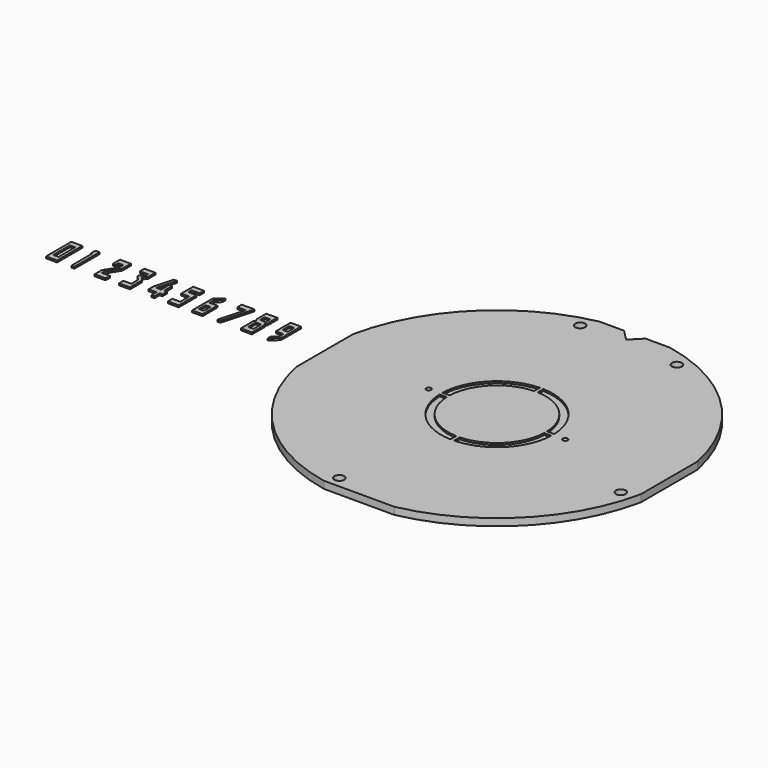
from build123d import *

# Parameters (mm, degrees)
F0_R      = 77.7875
F0_R_2    = 2.2
F0_R_3    = 1.1
F1_DEPTH  = 3.175
F3_DEPTH  = 3.175
F5_DEPTH  = 0.79375
F8_DEPTH  = 0.79375
F9_W      = 4.8782229424
F9_H      = 13.9600409893
F9_W_2    = 2.3128390312
F9_H_2    = 9.185263305
F10_DEPTH = 0.79375
F12_DEPTH = 0.79375
F14_DEPTH = 0.79375
F16_DEPTH = 0.79375
F18_DEPTH = 0.79375
F19_W     = 2.1891148112
F19_H     = 3.5902124946
F20_DEPTH = 0.79375
F22_DEPTH = 0.79375
F23_W     = 2.3770481348
F23_H     = 4.2385872221
F23_H_2   = 2.5488804094
F24_DEPTH = 0.79375
F25_W     = 2.229526639
F25_H     = 3.6757132038
F26_DEPTH = 0.79375
F27_W     = 165.1
F27_H     = 165.1
F27_W_2   = 152.4
F27_H_2   = 152.4
F28_DEPTH = 25.4


# Not quite as in the source:
# - a length typed as a fraction of an inch, garbled in the dataset ("3 / 203.2 mm" for 3/8 in), is restored


with BuildPart() as f1:
    # F0 (on Top) → F1 (new body)
    with BuildSketch(Plane.XY):
        Circle(F0_R)
        with Locations((-12.7, -71.2266277455)):
            Circle(F0_R_2, mode=Mode.SUBTRACT)
        with Locations((69.85, -18.854707635)):
            Circle(F0_R_2, mode=Mode.SUBTRACT)
        with Locations((-30.2125, 0)):
            Circle(F0_R_3, mode=Mode.SUBTRACT)
        with Locations((-19.05, 69.7969913392)):
            Circle(F0_R_2, mode=Mode.SUBTRACT)
        with Locations((30.2125, 0)):
            Circle(F0_R_3, mode=Mode.SUBTRACT)
        with Locations((25.4, 67.7448337514)):
            Circle(F0_R_2, mode=Mode.SUBTRACT)
    extrude(amount=F1_DEPTH)

    # F2 (on face) → F3 (cut, through all)
    with BuildSketch(Plane.XY.offset(3.175)):
        with BuildLine():
            Line((0, 71.4375), (6.1096910009, 77.5471910009))
            ThreePointArc((6.1096910009, 77.5471910009), (0, 77.7875), (-6.1096910009, 77.5471910009))
            Line((-6.1096910009, 77.5471910009), (0, 71.4375))
        make_face()
    extrude(amount=-F3_DEPTH, mode=Mode.SUBTRACT)

    # F4 (on face) → F5 (cut)
    with BuildSketch(Plane.XY.offset(3.175)):
        with BuildLine():
            ThreePointArc((-21.537278253, 0.79375), (-15.2394946375, 15.2394946375), (-0.79375, 21.537278253))
            Line((-0.79375, 21.537278253), (-0.79375, 24.7141567638))
            ThreePointArc((-0.79375, 24.7141567638), (-17.4845586677, 17.4845586677), (-24.7141567638, 0.79375))
            Line((-24.7141567638, 0.79375), (-21.537278253, 0.79375))
        make_face()
        with BuildLine():
            ThreePointArc((24.7141567638, 0.79375), (17.4845586677, 17.4845586677), (0.79375, 24.7141567638))
            Line((0.79375, 24.7141567638), (0.79375, 21.537278253))
            ThreePointArc((0.79375, 21.537278253), (15.2394946375, 15.2394946375), (21.537278253, 0.79375))
            Line((21.537278253, 0.79375), (24.7141567638, 0.79375))
        make_face()
        with BuildLine():
            Line((-0.79375, -24.7141567638), (-0.79375, -21.537278253))
            ThreePointArc((-0.79375, -21.537278253), (-15.2394946375, -15.2394946375), (-21.537278253, -0.79375))
            Line((-21.537278253, -0.79375), (-24.7141567638, -0.79375))
            ThreePointArc((-24.7141567638, -0.79375), (-17.4845586677, -17.4845586677), (-0.79375, -24.7141567638))
        make_face()
        with BuildLine():
            ThreePointArc((21.537278253, -0.79375), (15.2394946375, -15.2394946375), (0.79375, -21.537278253))
            Line((0.79375, -21.537278253), (0.79375, -24.7141567638))
            ThreePointArc((0.79375, -24.7141567638), (17.4845586677, -17.4845586677), (24.7141567638, -0.79375))
            Line((24.7141567638, -0.79375), (21.537278253, -0.79375))
        make_face()
    extrude(amount=-F5_DEPTH, mode=Mode.SUBTRACT)

    # F27 (on face) → F28 (cut)
    with BuildSketch(Plane.XY.offset(3.175)):
        Rectangle(F27_W, F27_H)
        Rectangle(F27_W_2, F27_H_2, mode=Mode.SUBTRACT)
    extrude(amount=-F28_DEPTH, mode=Mode.SUBTRACT)


with BuildPart() as f8:
    # F7 (on Top) → F8 (new body)
    with BuildSketch(Plane.XY):
        Polygon((-185.7131421566, -1.5020908322), (-185.7131421566, 12.45916076), (-187.0573009132, 12.45916076), (-187.5447928905, 11.9273522316), (-187.5447928905, 9.9914940074), (-187.0410889387, 9.9914940074), (-187.0410889387, -1.5020908322), align=None)
    extrude(amount=F8_DEPTH)


with BuildPart() as f10:
    # F9 (on Top) → F10 (new body)
    with BuildSketch(Plane.XY):
        with Locations((-195.7436352968, 5.4610763327)):
            Rectangle(F9_W, F9_H)
        with Locations((-195.7314908504, 5.4579324205)):
            Rectangle(F9_W_2, F9_H_2, mode=Mode.SUBTRACT)
    extrude(amount=F10_DEPTH)


with BuildPart() as f12:
    # F11 (on Top) → F12 (new body)
    with BuildSketch(Plane.XY):
        Polygon((-171.8911230564, 12.4986432493), (-176.7038702965, 12.4986432493), (-176.7038702965, 8.6026173085), (-175.4597574472, 8.6026173085), (-175.4597574472, 10.0104250014), (-173.2334643602, 10.0104250014), (-173.2334643602, 7.8823436052), (-176.7366081476, 2.4475506507), (-176.7366081476, -1.5139552997), (-171.8911230564, -1.5139552997), (-171.8911230564, 0.9415238746), (-175.4597574472, 0.9415238746), (-175.4597574472, 2.0546738524), (-171.8911230564, 7.6859053224), align=None)
    extrude(amount=F12_DEPTH)


with BuildPart() as f14:
    # F13 (on Top) → F14 (new body)
    with BuildSketch(Plane.XY):
        Polygon((-161.0794663429, 12.505360879), (-165.9247279167, 12.505360879), (-165.9247279167, 10.0249126554), (-162.3735427856, 10.0249126554), (-162.3735427856, 9.0121608227), (-164.5116657019, 6.7981919274), (-162.3735427856, 4.6379873529), (-162.3735427856, 4.5001455583), (-162.3735427856, 0.8887702134), (-165.9247279167, 0.8887702134), (-165.9247279167, -1.5188136604), (-161.0794663429, -1.5188136604), (-161.0794663429, 5.2519140216), (-162.6143008471, 6.8174446933), (-161.0794663429, 8.3221849054), align=None)
    extrude(amount=F14_DEPTH)


with BuildPart() as f16:
    # F15 (on Top) → F16 (new body)
    with BuildSketch(Plane.XY):
        Polygon((-151.4333486557, 12.4515779316), (-152.8201550245, 12.4515779316), (-155.1806926727, 3.8946401328), (-155.1806926727, 1.3865716755), (-151.639893651, 1.3865716755), (-151.639893651, -1.4755764278), (-150.3120958805, -1.4755764278), (-150.3120958805, 1.3865716755), (-149.1023153067, 1.3865716755), (-149.1023153067, 3.8946401328), (-150.3120958805, 3.8946401328), (-150.3120958805, 8.2911364734), (-151.639893651, 8.2911364734), (-151.639893651, 3.8946401328), (-153.7643671036, 3.8946401328), align=None)
    extrude(amount=F16_DEPTH)


with BuildPart() as f18:
    # F17 (on Top) → F18 (new body)
    with BuildSketch(Plane.XY):
        Polygon((-139.5121663809, 12.4827018008), (-144.3555355072, 12.4827018008), (-144.3555355072, 5.8832601644), (-140.7867372036, 5.8832601644), (-140.7867372036, 0.9549218812), (-144.3555355072, 0.9549218812), (-144.3555355072, -1.5092475805), (-139.5121663809, -1.5092475805), (-139.5121663809, 8.3474293351), (-143.1092917919, 8.3474293351), (-143.1092917919, 10.0468564779), (-139.5121663809, 10.0468564779), align=None)
    extrude(amount=F18_DEPTH)


with BuildPart() as f20:
    # F19 (on Top) → F20 (new body)
    with BuildSketch(Plane.XY):
        Polygon((-128.9858669043, 6.6911167463), (-132.407575967, 6.6911167463), (-132.407575967, 8.954399172), (-130.1615983248, 10.9099550173), (-130.1615983248, 12.5265857205), (-133.5712075233, 9.5578646287), (-133.5712075233, -1.5234014718), (-128.9858669043, -1.5234014718), align=None)
        with Locations((-131.3130185615, 2.5661735272)):
            Rectangle(F19_W, F19_H, mode=Mode.SUBTRACT)
    extrude(amount=F20_DEPTH)


with BuildPart() as f22:
    # F21 (on Top) → F22 (new body)
    with BuildSketch(Plane.XY):
        Polygon((-122.8491589427, 12.4853253365), (-122.8491589427, 10.0602889434), (-119.2461034646, 10.0602889434), (-122.4358007312, -1.5137457522), (-121.0854947567, -1.5137457522), (-117.2274798155, 12.4853253365), align=None)
    extrude(amount=F22_DEPTH)


with BuildPart() as f24:
    # F23 (on Top) → F24 (new body)
    with BuildSketch(Plane.XY):
        Polygon((-107.1394681931, 12.5098498538), (-112.0367571712, 12.5098498538), (-112.0367571712, 7.1543375961), (-111.3177399194, 6.3524427824), (-112.0367571712, 5.6067979562), (-112.0367571712, -1.5233105514), (-107.1394681931, -1.5233105514), (-107.1394681931, 5.6067979562), (-107.9127267003, 6.3524427824), (-107.1394681931, 7.1543375961), align=None)
        with Locations((-109.5594763756, 3.0016678502)):
            Rectangle(F23_W, F23_H, mode=Mode.SUBTRACT)
        with Locations((-109.5594763756, 8.8010861073)):
            Rectangle(F23_W, F23_H_2, mode=Mode.SUBTRACT)
    extrude(amount=F24_DEPTH)


with BuildPart() as f26:
    # F25 (on Top) → F26 (new body)
    with BuildSketch(Plane.XY):
        Polygon((-96.623711288, 12.4815516174), (-101.2360528111, 12.4815516174), (-101.2360528111, 4.2717433535), (-97.884865639, 4.2717433535), (-97.884865639, 1.917117224), (-100.1278907061, 0), (-100.1278907061, -1.6250308836), (-96.623711288, 1.3699970441), align=None)
        with Locations((-98.9496782422, 8.3592799492)):
            Rectangle(F25_W, F25_H, mode=Mode.SUBTRACT)
    extrude(amount=F26_DEPTH)


solid = Compound([f1.part, f8.part, f10.part, f12.part, f14.part, f16.part, f18.part, f20.part, f22.part, f24.part, f26.part])
